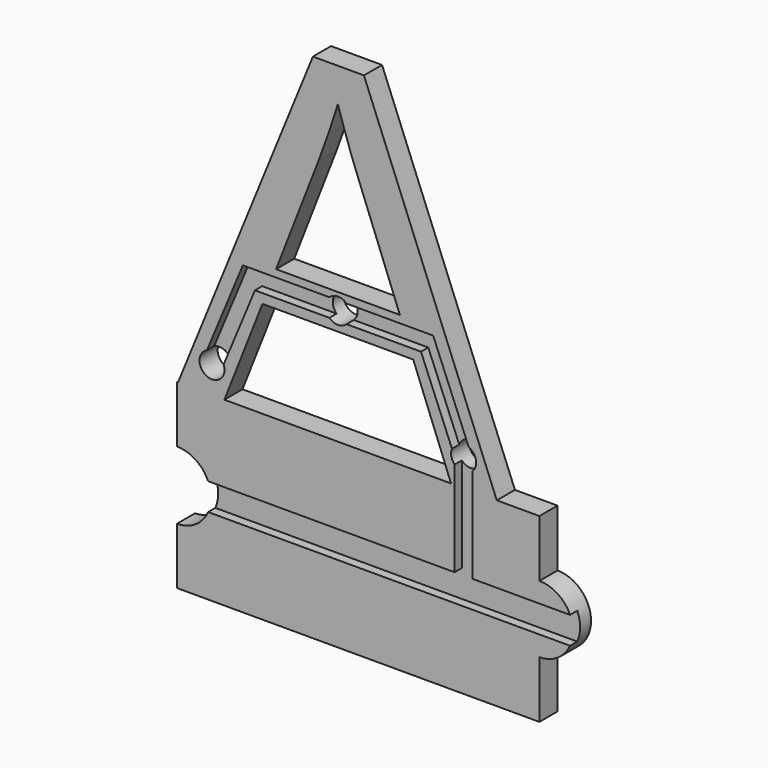
from build123d import *

# Parameters (mm, degrees)
F0_R     = 3.5052
F1_DEPTH = 6.35
F3_DEPTH = 2.54


with BuildPart() as f1:
    # F0 (on Front) → F1 (new body)
    with BuildSketch(Plane.XZ):
        Polygon((-11.3974893229, 44.2205731771), (-49.2346257812, -48.5394), (-36.2149429687, -48.5394), (-25.533746875, -21.4045270833), (16.7275536458, -21.4045270833), (27.3244799479, -48.5394), (40.1545557292, -48.5394), (2.9073078125, 44.2205731771), align=None)
        with Locations((-39.6848618984, -41.1395020783)):
            Circle(F0_R, mode=Mode.SUBTRACT)
        with Locations((30.8506265283, -41.1395020783)):
            Circle(F0_R, mode=Mode.SUBTRACT)
        with Locations((-4.3683550321, -16.2198841572)):
            Circle(F0_R, mode=Mode.SUBTRACT)
        with BuildLine():
            Line((-4.9929851562, 32.9073536458), (-4.4030966146, 34.7402216146))
            Line((-4.4030966146, 34.7402216146), (-2.6334309896, 29.2837526042))
            add(Edge.make_bspline(
                [(1.0533723958, 19.0028380208), (-0.7794955729, 23.5534067708), (-2.6334309896, 29.2837526042)],
                knots=[0, 0, 0, 1, 1, 1], degree=2))
            Line((1.0533723958, 19.0028380208), (12.9775479167, -11.6081638021))
            Line((12.9775479167, -11.6081638021), (-21.7205388021, -11.6081638021))
            Line((-21.7205388021, -11.6081638021), (-9.8806330729, 18.8764333333))
            add(Edge.make_bspline(
                [(-4.9929851562, 32.9073536458), (-6.6573135417, 27.4298171875), (-9.8806330729, 18.8764333333)],
                knots=[0, 0, 0, 1, 1, 1], degree=2))
        make_face(mode=Mode.SUBTRACT)
        with BuildLine():
            Line((-49.2346257812, -48.5394), (-49.5085026042, -48.5394))
            Line((-49.5085026042, -48.5394), (-49.5085026042, -64.4144))
            ThreePointArc((-49.5085026042, -64.4144), (-39.9835026042, -73.9394), (-49.5085026042, -83.4644))
            Line((-49.5085026042, -83.4644), (-49.5085026042, -99.3394))
            Line((-49.5085026042, -99.3394), (52.0914973958, -99.3394))
            Line((52.0914973958, -99.3394), (52.0914973958, -83.3374))
            ThreePointArc((52.0914973958, -83.3374), (61.4894973958, -73.9394), (52.0914973958, -64.5414))
            Line((52.0914973958, -64.5414), (52.0914973958, -48.5394))
            Line((52.0914973958, -48.5394), (40.1545557292, -48.5394))
            Line((40.1545557292, -48.5394), (27.3244799479, -48.5394))
            Line((27.3244799479, -48.5394), (-36.2149429687, -48.5394))
            Line((-36.2149429687, -48.5394), (-49.2346257812, -48.5394))
        make_face()
    extrude(amount=F1_DEPTH)

    # F2 (on face) → F3 (cut)
    with BuildSketch(Plane.XZ.offset(6.35)):
        with BuildLine():
            ThreePointArc((-6.7838939248, -18.7598839402), (-7.8735550321, -16.2198841572), (-6.7838939248, -13.6798843741))
            Line((-6.7838939248, -13.6798843741), (-31.0344029758, -13.6798843741))
            Line((-31.0344029758, -13.6798843741), (-41.1044888823, -37.9346485299))
            ThreePointArc((-41.1044888823, -37.9346485299), (-38.340810813, -37.902226415), (-36.4127835596, -39.882549261))
            Line((-36.4127835596, -39.882549261), (-27.6430815337, -18.7598839402))
            Line((-27.6430815337, -18.7598839402), (-6.7838939248, -18.7598839402))
        make_face()
        with BuildLine():
            ThreePointArc((27.5828955219, -39.8712903019), (29.5177289249, -37.8976182095), (32.2812779405, -37.9395546449))
            Line((32.2812779405, -37.9395546449), (22.3069365793, -13.6798843741))
            Line((22.3069365793, -13.6798843741), (-1.9528161394, -13.6798843741))
            ThreePointArc((-1.9528161394, -13.6798843741), (-1.1470684904, -14.8379507085), (-0.8631550321, -16.2198841572))
            ThreePointArc((-0.8631550321, -16.2198841572), (-1.1470684904, -17.6018176059), (-1.9528161394, -18.7598839402))
            Line((-1.9528161394, -18.7598839402), (18.9029600028, -18.7598839402))
            Line((18.9029600028, -18.7598839402), (27.5828955219, -39.8712903019))
        make_face()
        with BuildLine():
            Line((33.3906265283, -70.1294), (33.3906265283, -43.5550407429))
            ThreePointArc((33.3906265283, -43.5550407429), (30.8506265283, -44.6447020783), (28.3106265283, -43.5550407429))
            Line((28.3106265283, -43.5550407429), (28.3106265283, -70.1294))
            Line((28.3106265283, -70.1294), (-40.7786959053, -70.1294))
            ThreePointArc((-40.7786959053, -70.1294), (-39.9835026042, -73.9394), (-40.7786959053, -77.7494))
            Line((-40.7786959053, -77.7494), (60.6825569347, -77.7494))
            ThreePointArc((60.6825569347, -77.7494), (61.4894973958, -73.9394), (60.6825569347, -70.1294))
            Line((60.6825569347, -70.1294), (33.3906265283, -70.1294))
        make_face()
    extrude(amount=-F3_DEPTH, mode=Mode.SUBTRACT)


solid = f1.part
